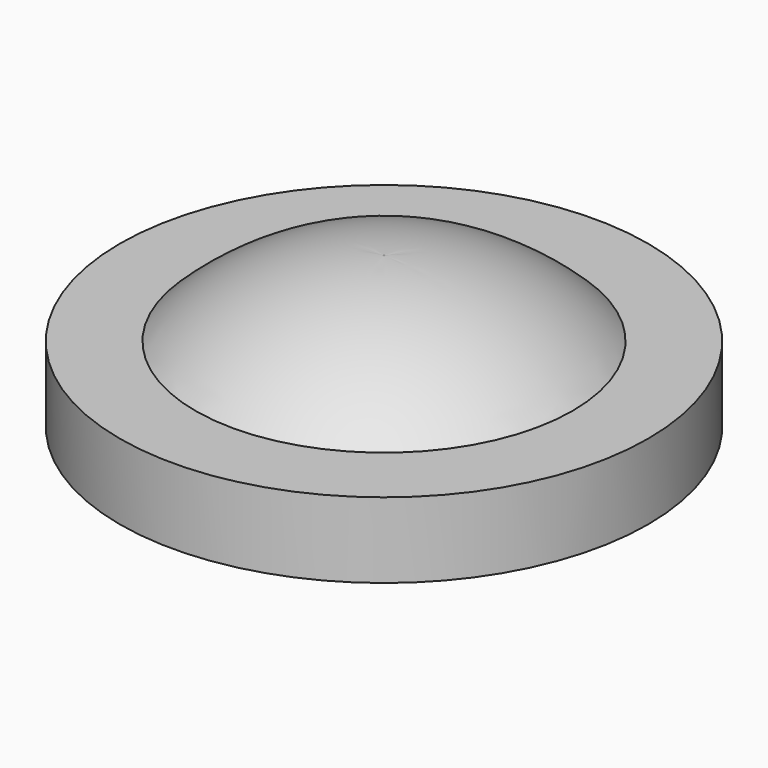
from build123d import *

# Parameters (mm, degrees)
F0_R     = 17.5
F1_DEPTH = 5
F2_R     = 12.5
F3_DEPTH = 5


# Not quite as in the source:
# - a fillet or chamfer that OpenCascade refuses, or shapes differently, is made with other operations: its cross-section is extruded or revolved along the edge and cut away or added


with BuildPart() as f1:
    # F0 (on Top) → F1 (new body)
    with BuildSketch(Plane.XY):
        Circle(F0_R)
    extrude(amount=F1_DEPTH)

    # F2 (on face) → F3 (join)
    with BuildSketch(Plane.XY.offset(5)):
        Circle(F2_R)
    extrude(amount=F3_DEPTH)

    # F4: fillet of radius 18 on 1 edges, made by hand

    # F4_s1 → F4_t2 (revolve, cut)
    with BuildSketch(Plane.XZ):
        with BuildLine():
            ThreePointArc((12.5, 5), (6.7583043345, 8.7032930885), (0.050100402, 10))
            Line((0.050100402, 10), (0.050100402, 10.36))
            Line((0.050100402, 10.36), (12.5, 10.36))
            Line((12.5, 10.36), (12.86, 10))
            ThreePointArc((12.86, 10), (12.86, 7.5), (12.748997992, 5.26))
            Line((12.748997992, 5.26), (12.5, 5))
        make_face()
    revolve(axis=Axis((0, 0, 10), (0, 0, 1)), mode=Mode.SUBTRACT)


solid = f1.part
